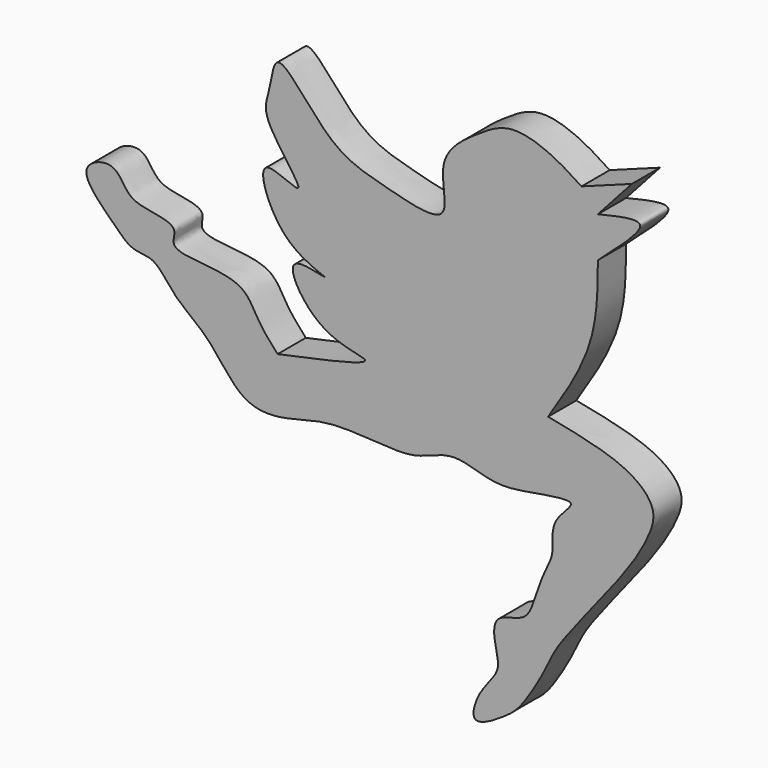
from build123d import *

# Parameters (mm, degrees)
F1_DEPTH = 3


with BuildPart() as f1:
    # F0 (on Front) → F1 (new body)
    with BuildSketch(Plane.XZ):
        with BuildLine():
            add(Edge.make_bspline(
                [(-2.4583407212, -0.9387893369), (-3.024112101, -0.3125586215), (-4.1330640857, 0.9148979442), (-5.1554360197, 3.2992855543), (-8.2577109297, 3.7518231514), (-11.7986873567, 3.9562154981), (-10.8820523568, 5.6551586921), (-12.6229603458, 6.247693459), (-15.315999481, 6.3953744354), (-16.1214771708, 9.2084322286), (-20.0168619315, 7.7469403625), (-16.4348146296, 4.3858640835), (-14.9096763531, 2.717360867), (-12.8034903879, 2.9512923233), (-11.2564726008, 0.3162128421), (-8.1642192374, -1.4569620139), (-5.6366346653, -5.782171544), (-1.6639945807, -5.7123551757), (2.0260628096, -4.2410968084), (8.2854144293, -5.1575498991), (10.3897632677, -4.3505708782), (12.7629271987, -3.4211792935), (15.9163275944, -4.8003006369), (18.878470836, -4.3406003478), (23.758674436, -3.4424946888), (20.5833092456, -5.7093836776), (21.1375367591, -8.1991364923), (20.3256954644, -9.5644173556), (19.4311703622, -11.9039628408), (18.8042825389, -14.238524747), (15.7594730051, -14.2173938905), (16.0097304788, -16.8272720908), (16.6128744696, -18.6430937651), (14.5862678652, -20.4291241442), (13.7016849232, -23.7435679152), (17.1599880674, -21.6476481949), (18.4130917332, -20.4613319605), (20.4135012758, -17.0905072069), (21.2051604651, -14.8895883579), (26.6442672206, -8.5043457259), (29.0228229475, -4.7255734803), (29.9094935065, -2.0250450932), (27.1712719561, 0.5621773403), (23.0298835059, 1.3712804026), (20.5461345613, 1.8565304345)],
                knots=[0, 0, 0, 0, 0.0223183973, 0.0437456398, 0.0688985616, 0.0927213027, 0.1071661769, 0.1240978569, 0.1467675231, 0.1680579867, 0.1893657062, 0.2167940554, 0.2386379801, 0.2569750139, 0.2801606546, 0.307161996, 0.3374507126, 0.3634276608, 0.3920866547, 0.4268369435, 0.4479230873, 0.4693503305, 0.4943624909, 0.5208560372, 0.5459071395, 0.5665532363, 0.5884766445, 0.6058484831, 0.628251547, 0.6490610711, 0.6703449254, 0.6905625398, 0.7093141047, 0.7324792265, 0.7527913136, 0.7758969033, 0.7965464522, 0.8230888703, 0.8456282197, 0.8859909385, 0.9167367705, 0.9381017064, 0.9628772275, 1, 1, 1, 1], degree=3))
            add(Edge.make_bspline(
                [(20.5461345613, 1.8565304345), (21.9843605456, 4.0877615411), (24.7378369306, 8.3594422288), (24.7652508293, 12.8195046032), (24.7783455998, 14.9499382824)],
                knots=[0, 0, 0, 0, 0.5223309675, 1, 1, 1, 1], degree=3))
            add(Edge.make_bspline(
                [(24.7783455998, 14.9499382824), (26.6874267886, 16.6217989258), (30.1772593082, 19.6779882987), (26.4614535575, 18.7905731041), (24.7783455998, 18.3886103332)],
                knots=[0, 0, 0, 0, 0.5470409191, 1, 1, 1, 1], degree=3))
            Line((24.7783455998, 18.3886103332), (27.6668481529, 21.598758176))
            Line((27.6668481529, 21.598758176), (23.3847144991, 20.0211293995))
            add(Edge.make_bspline(
                [(23.3847144991, 20.0211293995), (22.5338494252, 20.5791637074), (20.7976546345, 21.7178357343), (17.2504722248, 22.8214880736), (14.4564571643, 21.0489460918), (10.6854307395, 18.3554386667), (12.8440522505, 12.8765681684), (6.2419581214, 14.7424087726), (1.9232853652, 15.7514937162), (-2.7342242262, 22.7341263785), (-3.0219837282, 18.3915805656), (-4.1605211958, 16.4916585466), (1.2731668381, 10.4575548527), (-4.8138967458, 14.2916323506), (-2.4928932067, 7.7474018762), (0.2045257408, 6.6764107619), (1.5984182246, 6.1229756102)],
                knots=[0, 0, 0, 0, 0.0644146999, 0.1314385439, 0.1968319706, 0.2714811413, 0.3413548458, 0.4200475802, 0.5057778314, 0.5937833005, 0.6485754625, 0.7072372091, 0.7871471919, 0.8471291748, 0.9210039306, 1, 1, 1, 1], degree=3))
            add(Edge.make_bspline(
                [(1.5984182246, 6.1229756102), (0.3794385893, 6.3947330374), (-2.4552391583, 7.0266916932), (1.0076209648, 1.3792102604), (7.607088459, 1.1883117848), (1.2931039504, -0.1460062349), (-2.4583407212, -0.9387893369)],
                knots=[0, 0, 0, 0, 0.1936687603, 0.4503672655, 0.6734365138, 1, 1, 1, 1], degree=3))
        make_face()
        with BuildLine():
            add(Edge.make_bspline(
                [(22.6999428123, 19.3365197629), (22.3242155898, 19.5631626942), (21.4544289305, 20.0878278935), (19.2659041282, 21.4051754613), (16.6460371205, 21.4763759863), (13.5816483172, 20.043221821), (12.2892210529, 17.8095974256), (12.5681196065, 15.0871928348), (12.3230838562, 12.8978219278), (8.8639840954, 13.0449553336), (5.2066810805, 14.151426431), (1.707829216, 14.9353315218), (-1.170779148, 18.1401441424), (-1.5655897851, 20.4183641193), (-2.5929770673, 19.4536346829), (-2.5932049211, 17.9614670798), (-2.6339004563, 16.4813338584), (-0.3224472186, 13.7380850634), (0.6135356219, 11.7639540273), (-0.7167249297, 10.8530067604), (-3.3318702702, 12.7121257392), (-2.5667672816, 10.6745545783), (-1.5094169541, 8.4459250214), (2.1106983207, 7.2381496114), (2.7645327104, 6.2696114421), (3.0224460643, 5.8875591494)],
                knots=[0, 0, 0, 0, 0.0345222802, 0.0799170701, 0.1264160139, 0.1782976735, 0.2232215976, 0.270993781, 0.3087962495, 0.3578588003, 0.4157076401, 0.4703647639, 0.5300860598, 0.5673107508, 0.5934188369, 0.6284721036, 0.6631450996, 0.7179951551, 0.7579670519, 0.788326596, 0.8317622624, 0.8624300866, 0.909423256, 0.9642708426, 1, 1, 1, 1], degree=3))
            Line((22.6999428123, 19.3365197629), (26.0433372777, 20.5682971304))
            Line((26.0433372777, 20.5682971304), (24.0020574897, 18.3859034087))
            add(Edge.make_bspline(
                [(17.7613161504, 1.2181339553), (18.3459469112, 2.0293237663), (19.6496885009, 3.8382978482), (22.3270533593, 7.85048253), (23.2824396662, 12.4940733784), (23.1220059605, 15.9857519702), (25.3202795702, 16.5504719842), (27.8645173763, 18.1667392321), (26.1450777549, 18.0905903306), (24.3352004071, 17.6754938561), (24.0907529204, 18.1967651202), (24.0020574897, 18.3859034087)],
                knots=[0, 0, 0, 0, 0.1275196806, 0.284372158, 0.4427790882, 0.5660647269, 0.6719001823, 0.7765117048, 0.8460306235, 0.9441336855, 1, 1, 1, 1], degree=3))
            add(Edge.make_bspline(
                [(24.4001187384, -3.3008425962), (24.3409545974, -3.6554720505), (24.2018944746, -4.4889974695), (22.2223315181, -5.7543203865), (22.4832289942, -8.9296135449), (20.3988923072, -12.2579807717), (20.019356702, -14.9437682798), (17.1257288874, -14.9016519593), (16.6563720182, -16.1673443115), (17.6416824742, -18.42647415), (15.9248500213, -20.4490406816), (14.6742381442, -22.1678172602), (17.3676591915, -20.8599894053), (19.2062636839, -16.9301620982), (22.395345056, -11.5365370821), (25.0840863289, -7.2209170092), (27.9509062353, -4.1529344918), (28.0643595577, -0.9185538348), (21.4065022533, 0.3237566534), (18.8864877652, 0.9420635642), (17.7613161504, 1.2181339553)],
                knots=[0, 0, 0, 0, 0.0342545275, 0.0805122615, 0.1365401346, 0.2013155909, 0.2511031186, 0.3006525471, 0.3335558205, 0.3817053118, 0.4353696827, 0.4714452042, 0.5144946797, 0.5840870765, 0.6661694447, 0.7406786923, 0.8061006005, 0.8549144632, 0.935220163, 1, 1, 1, 1], degree=3))
            add(Edge.make_bspline(
                [(3.0224460643, 5.8875591494), (2.6605674816, 5.7112317822), (1.9018445059, 5.3415397609), (0.613870925, 5.8961917239), (-0.4468114988, 6.1732975767), (-0.5991275153, 5.4758399813), (0.4148661064, 3.8408525846), (1.4386873446, 2.6784537478), (4.8974896565, 1.8585546414), (6.4785231574, 1.348921805), (5.2639700351, -0.4949434958), (1.2648465469, -0.947879165), (-1.7303055212, -1.9880112414), (-4.1498291031, -1.7144645068), (-5.6092074984, 1.0551090331), (-6.2769311874, 2.7645892095), (-9.7310375403, 2.9240494367), (-12.6399330685, 3.4799357512), (-11.5045287811, 6.0347840809), (-15.3225081475, 4.9080547315), (-15.9460754267, 8.0552125685), (-18.1680344995, 7.8080997394), (-17.0845579282, 5.84994772), (-14.9938162063, 4.0224657221), (-13.0229620708, 3.6056954547), (-10.9976580316, 1.8051812839), (-7.6082138342, 0.7572762248), (-5.7361926252, -3.4870897446), (-1.7411166, -4.7228943753), (2.0828785576, -2.7694583145), (7.3146646675, -4.390656531), (11.2428375966, -1.4464033457), (15.8676265775, -3.939807471), (20.2513749856, -2.6018494682), (23.0434376746, -2.7898009003), (24.001643128, -3.1507427259), (24.4001187384, -3.3008425962)],
                knots=[0, 0, 0, 0, 0.0203763207, 0.0427214636, 0.0607192903, 0.0733745539, 0.0987475418, 0.1228836, 0.158441793, 0.1793079016, 0.202042841, 0.23992768, 0.2739458096, 0.3013412751, 0.3334163755, 0.3575495119, 0.3920799182, 0.4213661423, 0.4439054505, 0.4740907577, 0.5042622531, 0.5252665904, 0.5491831564, 0.5810702351, 0.6073180449, 0.6375310291, 0.6721804859, 0.7112858235, 0.7471787688, 0.7851429286, 0.8275064884, 0.8664485522, 0.9072035833, 0.9471463298, 0.9780204773, 1, 1, 1, 1], degree=3))
        make_face(mode=Mode.SUBTRACT)
        with BuildLine():
            Line((26.0433372777, 20.5682971304), (22.6999428123, 19.3365197629))
            add(Edge.make_bspline(
                [(22.6999428123, 19.3365197629), (22.3242155898, 19.5631626942), (21.4544289305, 20.0878278935), (19.2659041282, 21.4051754613), (16.6460371205, 21.4763759863), (13.5816483172, 20.043221821), (12.2892210529, 17.8095974256), (12.5681196065, 15.0871928348), (12.3230838562, 12.8978219278), (8.8639840954, 13.0449553336), (5.2066810805, 14.151426431), (1.707829216, 14.9353315218), (-1.170779148, 18.1401441424), (-1.5655897851, 20.4183641193), (-2.5929770673, 19.4536346829), (-2.5932049211, 17.9614670798), (-2.6339004563, 16.4813338584), (-0.3224472186, 13.7380850634), (0.6135356219, 11.7639540273), (-0.7167249297, 10.8530067604), (-3.3318702702, 12.7121257392), (-2.5667672816, 10.6745545783), (-1.5094169541, 8.4459250214), (2.1106983207, 7.2381496114), (2.7645327104, 6.2696114421), (3.0224460643, 5.8875591494)],
                knots=[0, 0, 0, 0, 0.0345222802, 0.0799170701, 0.1264160139, 0.1782976735, 0.2232215976, 0.270993781, 0.3087962495, 0.3578588003, 0.4157076401, 0.4703647639, 0.5300860598, 0.5673107508, 0.5934188369, 0.6284721036, 0.6631450996, 0.7179951551, 0.7579670519, 0.788326596, 0.8317622624, 0.8624300866, 0.909423256, 0.9642708426, 1, 1, 1, 1], degree=3))
            add(Edge.make_bspline(
                [(3.0224460643, 5.8875591494), (2.6605674816, 5.7112317822), (1.9018445059, 5.3415397609), (0.613870925, 5.8961917239), (-0.4468114988, 6.1732975767), (-0.5991275153, 5.4758399813), (0.4148661064, 3.8408525846), (1.4386873446, 2.6784537478), (4.8974896565, 1.8585546414), (6.4785231574, 1.348921805), (5.2639700351, -0.4949434958), (1.2648465469, -0.947879165), (-1.7303055212, -1.9880112414), (-4.1498291031, -1.7144645068), (-5.6092074984, 1.0551090331), (-6.2769311874, 2.7645892095), (-9.7310375403, 2.9240494367), (-12.6399330685, 3.4799357512), (-11.5045287811, 6.0347840809), (-15.3225081475, 4.9080547315), (-15.9460754267, 8.0552125685), (-18.1680344995, 7.8080997394), (-17.0845579282, 5.84994772), (-14.9938162063, 4.0224657221), (-13.0229620708, 3.6056954547), (-10.9976580316, 1.8051812839), (-7.6082138342, 0.7572762248), (-5.7361926252, -3.4870897446), (-1.7411166, -4.7228943753), (2.0828785576, -2.7694583145), (7.3146646675, -4.390656531), (11.2428375966, -1.4464033457), (15.8676265775, -3.939807471), (20.2513749856, -2.6018494682), (23.0434376746, -2.7898009003), (24.001643128, -3.1507427259), (24.4001187384, -3.3008425962)],
                knots=[0, 0, 0, 0, 0.0203763207, 0.0427214636, 0.0607192903, 0.0733745539, 0.0987475418, 0.1228836, 0.158441793, 0.1793079016, 0.202042841, 0.23992768, 0.2739458096, 0.3013412751, 0.3334163755, 0.3575495119, 0.3920799182, 0.4213661423, 0.4439054505, 0.4740907577, 0.5042622531, 0.5252665904, 0.5491831564, 0.5810702351, 0.6073180449, 0.6375310291, 0.6721804859, 0.7112858235, 0.7471787688, 0.7851429286, 0.8275064884, 0.8664485522, 0.9072035833, 0.9471463298, 0.9780204773, 1, 1, 1, 1], degree=3))
            add(Edge.make_bspline(
                [(24.4001187384, -3.3008425962), (24.3409545974, -3.6554720505), (24.2018944746, -4.4889974695), (22.2223315181, -5.7543203865), (22.4832289942, -8.9296135449), (20.3988923072, -12.2579807717), (20.019356702, -14.9437682798), (17.1257288874, -14.9016519593), (16.6563720182, -16.1673443115), (17.6416824742, -18.42647415), (15.9248500213, -20.4490406816), (14.6742381442, -22.1678172602), (17.3676591915, -20.8599894053), (19.2062636839, -16.9301620982), (22.395345056, -11.5365370821), (25.0840863289, -7.2209170092), (27.9509062353, -4.1529344918), (28.0643595577, -0.9185538348), (21.4065022533, 0.3237566534), (18.8864877652, 0.9420635642), (17.7613161504, 1.2181339553)],
                knots=[0, 0, 0, 0, 0.0342545275, 0.0805122615, 0.1365401346, 0.2013155909, 0.2511031186, 0.3006525471, 0.3335558205, 0.3817053118, 0.4353696827, 0.4714452042, 0.5144946797, 0.5840870765, 0.6661694447, 0.7406786923, 0.8061006005, 0.8549144632, 0.935220163, 1, 1, 1, 1], degree=3))
            add(Edge.make_bspline(
                [(17.7613161504, 1.2181339553), (18.3459469112, 2.0293237663), (19.6496885009, 3.8382978482), (22.3270533593, 7.85048253), (23.2824396662, 12.4940733784), (23.1220059605, 15.9857519702), (25.3202795702, 16.5504719842), (27.8645173763, 18.1667392321), (26.1450777549, 18.0905903306), (24.3352004071, 17.6754938561), (24.0907529204, 18.1967651202), (24.0020574897, 18.3859034087)],
                knots=[0, 0, 0, 0, 0.1275196806, 0.284372158, 0.4427790882, 0.5660647269, 0.6719001823, 0.7765117048, 0.8460306235, 0.9441336855, 1, 1, 1, 1], degree=3))
            Line((24.0020574897, 18.3859034087), (26.0433372777, 20.5682971304))
        make_face()
    extrude(amount=F1_DEPTH)


solid = f1.part
